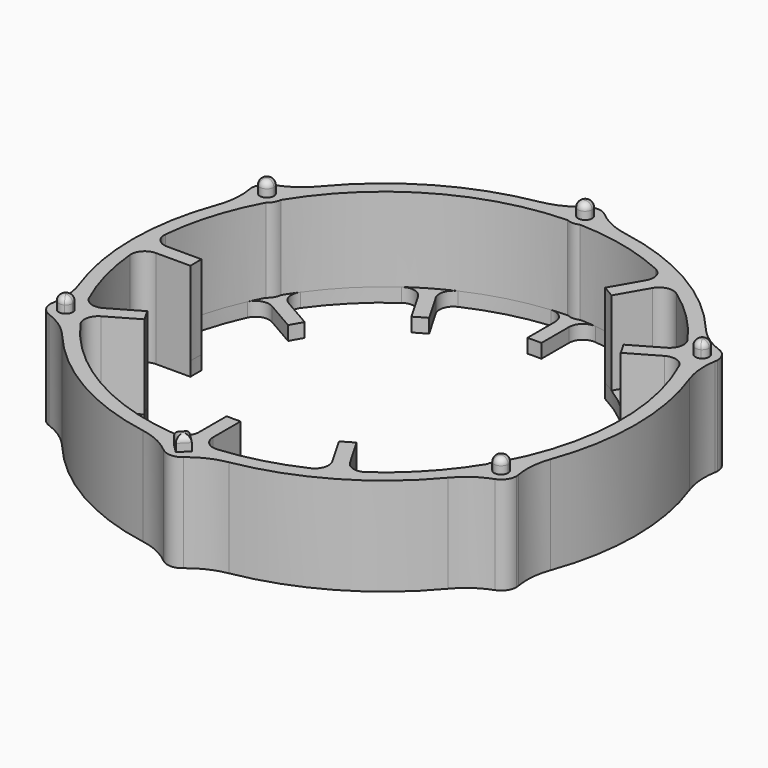
from build123d import *

# Parameters (mm, degrees)
F1_R         = 18
F1_R_2       = 17
F2_DEPTH     = 7
F3_DEPTH     = 7
F4_DEPTH     = 1
F6_DEPTH     = 7
F7_R         = 1
F8_R         = 5
F9_DEPTH     = 8
F10_R        = 0.44999
F11_DEPTH    = 1.8
F12_R        = 13.47
F13_DEPTH    = 1
F14_DEPTH    = 1
F15_T1_DEPTH = 3.7395798703
F15_T3_DEPTH = 1


# Not quite as in the source:
# - a fillet or chamfer that OpenCascade refuses, or shapes differently, is made with other operations: its cross-section is extruded or revolved along the edge and cut away or added
# - a fillet or chamfer is up to 0.001 mm smaller than in the source, because OpenCascade refuses the exact size
# - after a boolean that leaves OpenCascade's solid faulty, fix() repairs it


with BuildPart() as f2:
    # F1 (on Top) → F2 (new body)
    with BuildSketch(Plane.XY):
        Circle(F1_R)
        Circle(F1_R_2, mode=Mode.SUBTRACT)
    extrude(amount=F2_DEPTH)

    # F0 (on Top) → F3 (join)
    with BuildSketch(Plane.XY):
        with BuildLine():
            Line((7.1633711619, 11.4073228059), (8.9293354359, 14.4660626528))
            ThreePointArc((8.9293354359, 14.4660626528), (8.5, 14.7224318643), (8.0633100321, 14.9660626528))
            Line((8.0633100321, 14.9660626528), (6.2973457581, 11.9073228059))
            ThreePointArc((6.2973457581, 11.9073228059), (6.735, 11.665362189), (7.1633711619, 11.4073228059))
        make_face()
        with BuildLine():
            ThreePointArc((-0.5, -16.992645468), (0, -17), (0.5, -16.992645468))
            Line((0.5, -16.992645468), (0.5, -13.46071692))
            ThreePointArc((0.5, -13.46071692), (0, -13.47), (-0.5, -13.46071692))
            Line((-0.5, -13.46071692), (-0.5, -16.992645468))
        make_face()
        with BuildLine():
            ThreePointArc((-14.9660626528, -8.0633100321), (-14.7224318643, -8.5), (-14.4660626528, -8.9293354359))
            Line((-14.4660626528, -8.9293354359), (-11.4073228059, -7.1633711619))
            ThreePointArc((-11.4073228059, -7.1633711619), (-11.665362189, -6.735), (-11.9073228059, -6.2973457581))
            Line((-11.9073228059, -6.2973457581), (-14.9660626528, -8.0633100321))
        make_face()
        with BuildLine():
            Line((11.9073228059, 6.2973457581), (14.9660626528, 8.0633100321))
            ThreePointArc((14.9660626528, 8.0633100321), (14.7224318643, 8.5), (14.4660626528, 8.9293354359))
            Line((14.4660626528, 8.9293354359), (11.4073228059, 7.1633711619))
            ThreePointArc((11.4073228059, 7.1633711619), (11.665362189, 6.735), (11.9073228059, 6.2973457581))
        make_face()
        with BuildLine():
            ThreePointArc((8.0633100321, -14.9660626528), (8.5, -14.7224318643), (8.9293354359, -14.4660626528))
            Line((8.9293354359, -14.4660626528), (7.1633711619, -11.4073228059))
            ThreePointArc((7.1633711619, -11.4073228059), (6.735, -11.665362189), (6.2973457581, -11.9073228059))
            Line((6.2973457581, -11.9073228059), (8.0633100321, -14.9660626528))
        make_face()
        with BuildLine():
            Line((-13.46071692, 0.5), (-16.992645468, 0.5))
            ThreePointArc((-16.992645468, 0.5), (-17, 0), (-16.992645468, -0.5))
            Line((-16.992645468, -0.5), (-13.46071692, -0.5))
            ThreePointArc((-13.46071692, -0.5), (-13.47, 0), (-13.46071692, 0.5))
        make_face()
    extrude(amount=F3_DEPTH)

    # F1 (on Top) → F4 (join)
    with BuildSketch(Plane.XY):
        Circle(F1_R)
        Circle(F1_R_2, mode=Mode.SUBTRACT)
        Circle(F1_R_2)
    extrude(amount=F4_DEPTH)

    # F5 (on Top) → F6 (join)
    with BuildSketch(Plane.XY):
        with BuildLine():
            ThreePointArc((-14.4884572681, 9), (-14.6275367743, 9.5353800561), (-15.0096060035, 9.935377578))
            ThreePointArc((-15.0096060035, 9.935377578), (-15.1731450826, 9.6837837802), (-15.3324673166, 9.4294987133))
            ThreePointArc((-15.3324673166, 9.4294987133), (-15.153718855, 9.2469868663), (-15.0884572681, 9))
            ThreePointArc((-15.0884572681, 9), (-15.3354561915, 8.5687338928), (-15.832419089, 8.5635568422))
            ThreePointArc((-15.832419089, 8.5635568422), (-15.9729752997, 8.2984372068), (-16.1090923805, 8.0310113108))
            ThreePointArc((-16.1090923805, 8.0310113108), (-15.0239657375, 8.0558870238), (-14.4884572681, 9))
        make_face()
        with BuildLine():
            ThreePointArc((-15.3324673166, 9.4294987133), (-15.1731450826, 9.6837837802), (-15.0096060035, 9.935377578))
            ThreePointArc((-15.0096060035, 9.935377578), (-16.5410852123, 9.55), (-16.1090923805, 8.0310113108))
            ThreePointArc((-16.1090923805, 8.0310113108), (-15.9729752997, 8.2984372068), (-15.832419089, 8.5635568422))
            ThreePointArc((-15.832419089, 8.5635568422), (-16.02146997, 9.25), (-15.3324673166, 9.4294987133))
        make_face()
        with BuildLine():
            ThreePointArc((-1.099486377, 17.9663888889), (0, 16.9), (1.099486377, 17.9663888889))
            ThreePointArc((1.099486377, 17.9663888889), (0.7998302171, 17.982220987), (0.4999517724, 17.9930555556))
            ThreePointArc((0.4999517724, 17.9930555556), (0, 17.5), (-0.4999517724, 17.9930555556))
            ThreePointArc((-0.4999517724, 17.9930555556), (-0.7998302171, 17.982220987), (-1.099486377, 17.9663888889))
        make_face()
        with BuildLine():
            ThreePointArc((0.4999517724, 17.9930555556), (0.7998302171, 17.982220987), (1.099486377, 17.9663888889))
            ThreePointArc((1.099486377, 17.9663888889), (1.0998715868, 17.9831924823), (1.1, 18))
            ThreePointArc((1.1, 18), (-0.0168075177, 19.0998715868), (-1.099486377, 17.9663888889))
            ThreePointArc((-1.099486377, 17.9663888889), (-0.7998302171, 17.982220987), (-0.4999517724, 17.9930555556))
            ThreePointArc((-0.4999517724, 17.9930555556), (-0.003472306, 18.4999879429), (0.5, 18))
            ThreePointArc((0.5, 18), (0.4999879429, 17.996527694), (0.4999517724, 17.9930555556))
        make_face()
        with BuildLine():
            ThreePointArc((15.832419089, 8.5635568422), (15.9729752997, 8.2984372068), (16.1090923805, 8.0310113108))
            ThreePointArc((16.1090923805, 8.0310113108), (16.5325702443, 8.4355084694), (16.6884572681, 9))
            ThreePointArc((16.6884572681, 9), (16.1238373242, 9.9609204939), (15.0096060035, 9.935377578))
            ThreePointArc((15.0096060035, 9.935377578), (15.1731450826, 9.6837837802), (15.3324673166, 9.4294987133))
            ThreePointArc((15.3324673166, 9.4294987133), (15.8354441344, 9.4347384132), (16.0884572681, 9))
            ThreePointArc((16.0884572681, 9), (16.0197233753, 8.7469989234), (15.832419089, 8.5635568422))
        make_face()
        with BuildLine():
            ThreePointArc((15.0096060035, 9.935377578), (14.635829324, 8.45), (16.1090923805, 8.0310113108))
            ThreePointArc((16.1090923805, 8.0310113108), (15.9729752997, 8.2984372068), (15.832419089, 8.5635568422))
            ThreePointArc((15.832419089, 8.5635568422), (15.1554445662, 8.75), (15.3324673166, 9.4294987133))
            ThreePointArc((15.3324673166, 9.4294987133), (15.1731450826, 9.6837837802), (15.0096060035, 9.935377578))
        make_face()
        with BuildLine():
            ThreePointArc((-15.3324673166, -9.4294987133), (-15.1731450826, -9.6837837802), (-15.0096060035, -9.935377578))
            ThreePointArc((-15.0096060035, -9.935377578), (-14.6275367743, -9.5353800561), (-14.4884572681, -9))
            ThreePointArc((-14.4884572681, -9), (-15.0239657375, -8.0558870238), (-16.1090923805, -8.0310113108))
            ThreePointArc((-16.1090923805, -8.0310113108), (-15.9729752997, -8.2984372068), (-15.832419089, -8.5635568422))
            ThreePointArc((-15.832419089, -8.5635568422), (-15.3354561915, -8.5687338928), (-15.0884572681, -9))
            ThreePointArc((-15.0884572681, -9), (-15.153718855, -9.2469868663), (-15.3324673166, -9.4294987133))
        make_face()
        with BuildLine():
            ThreePointArc((-16.1090923805, -8.0310113108), (-16.5410852123, -9.55), (-15.0096060035, -9.935377578))
            ThreePointArc((-15.0096060035, -9.935377578), (-15.1731450826, -9.6837837802), (-15.3324673166, -9.4294987133))
            ThreePointArc((-15.3324673166, -9.4294987133), (-16.02146997, -9.25), (-15.832419089, -8.5635568422))
            ThreePointArc((-15.832419089, -8.5635568422), (-15.9729752997, -8.2984372068), (-16.1090923805, -8.0310113108))
        make_face()
        with BuildLine():
            ThreePointArc((0.6255239257, -17.9891278226), (0.8625800837, -17.9793202207), (1.099486377, -17.9663888889))
            ThreePointArc((1.099486377, -17.9663888889), (0, -16.9), (-1.099486377, -17.9663888889))
            ThreePointArc((-1.099486377, -17.9663888889), (-0.8625800837, -17.9793202207), (-0.6255239257, -17.9891278226))
            Line((-0.6255239257, -17.9891278226), (0, -17.3636038969))
            Line((0, -17.3636038969), (0.6255239257, -17.9891278226))
        make_face()
        with BuildLine():
            ThreePointArc((1.1, -18), (1.0998715868, -17.9831924823), (1.099486377, -17.9663888889))
            ThreePointArc((1.099486377, -17.9663888889), (0.8625800837, -17.9793202207), (0.6255239257, -17.9891278226))
            Line((0.6255239257, -17.9891278226), (0.6363961031, -18))
            Line((0.6363961031, -18), (0, -18.6363961031))
            Line((0, -18.6363961031), (-0.6363961031, -18))
            Line((-0.6363961031, -18), (-0.6255239257, -17.9891278226))
            ThreePointArc((-0.6255239257, -17.9891278226), (-0.8625800837, -17.9793202207), (-1.099486377, -17.9663888889))
            ThreePointArc((-1.099486377, -17.9663888889), (-0.0168075177, -19.0998715868), (1.1, -18))
        make_face()
        with BuildLine():
            ThreePointArc((16.6884572681, -9), (16.5325702443, -8.4355084694), (16.1090923805, -8.0310113108))
            ThreePointArc((16.1090923805, -8.0310113108), (15.9729752997, -8.2984372068), (15.832419089, -8.5635568422))
            ThreePointArc((15.832419089, -8.5635568422), (16.0197233753, -8.7469989234), (16.0884572681, -9))
            ThreePointArc((16.0884572681, -9), (15.8354441344, -9.4347384132), (15.3324673166, -9.4294987133))
            ThreePointArc((15.3324673166, -9.4294987133), (15.1731450826, -9.6837837802), (15.0096060035, -9.935377578))
            ThreePointArc((15.0096060035, -9.935377578), (16.1238373242, -9.9609204939), (16.6884572681, -9))
        make_face()
        with BuildLine():
            ThreePointArc((15.832419089, -8.5635568422), (15.9729752997, -8.2984372068), (16.1090923805, -8.0310113108))
            ThreePointArc((16.1090923805, -8.0310113108), (14.635829324, -8.45), (15.0096060035, -9.935377578))
            ThreePointArc((15.0096060035, -9.935377578), (15.1731450826, -9.6837837802), (15.3324673166, -9.4294987133))
            ThreePointArc((15.3324673166, -9.4294987133), (15.1554445662, -8.75), (15.832419089, -8.5635568422))
        make_face()
        with BuildLine():
            ThreePointArc((-15.0884572681, 9), (-15.153718855, 9.2469868663), (-15.3324673166, 9.4294987133))
            ThreePointArc((-15.3324673166, 9.4294987133), (-15.5884572681, 9), (-15.832419089, 8.5635568422))
            ThreePointArc((-15.832419089, 8.5635568422), (-15.3354561915, 8.5687338928), (-15.0884572681, 9))
        make_face()
        with BuildLine():
            ThreePointArc((-15.832419089, 8.5635568422), (-15.5884572681, 9), (-15.3324673166, 9.4294987133))
            ThreePointArc((-15.3324673166, 9.4294987133), (-16.02146997, 9.25), (-15.832419089, 8.5635568422))
        make_face()
        with BuildLine():
            ThreePointArc((-0.4999517724, 17.9930555556), (0, 18), (0.4999517724, 17.9930555556))
            ThreePointArc((0.4999517724, 17.9930555556), (0.4999879429, 17.996527694), (0.5, 18))
            ThreePointArc((0.5, 18), (-0.003472306, 18.4999879429), (-0.4999517724, 17.9930555556))
        make_face()
        with BuildLine():
            ThreePointArc((-0.4999517724, 17.9930555556), (0, 17.5), (0.4999517724, 17.9930555556))
            ThreePointArc((0.4999517724, 17.9930555556), (0, 18), (-0.4999517724, 17.9930555556))
        make_face()
        with BuildLine():
            ThreePointArc((15.3324673166, 9.4294987133), (15.5884572681, 9), (15.832419089, 8.5635568422))
            ThreePointArc((15.832419089, 8.5635568422), (16.0197233753, 8.7469989234), (16.0884572681, 9))
            ThreePointArc((16.0884572681, 9), (15.8354441344, 9.4347384132), (15.3324673166, 9.4294987133))
        make_face()
        with BuildLine():
            ThreePointArc((15.3324673166, 9.4294987133), (15.1554445662, 8.75), (15.832419089, 8.5635568422))
            ThreePointArc((15.832419089, 8.5635568422), (15.5884572681, 9), (15.3324673166, 9.4294987133))
        make_face()
        with BuildLine():
            ThreePointArc((16.0884572681, -9), (16.0197233753, -8.7469989234), (15.832419089, -8.5635568422))
            ThreePointArc((15.832419089, -8.5635568422), (15.5884572681, -9), (15.3324673166, -9.4294987133))
            ThreePointArc((15.3324673166, -9.4294987133), (15.8354441344, -9.4347384132), (16.0884572681, -9))
        make_face()
        with BuildLine():
            ThreePointArc((15.3324673166, -9.4294987133), (15.5884572681, -9), (15.832419089, -8.5635568422))
            ThreePointArc((15.832419089, -8.5635568422), (15.1554445662, -8.75), (15.3324673166, -9.4294987133))
        make_face()
        with BuildLine():
            Line((0.6363961031, -18), (0.6255239257, -17.9891278226))
            ThreePointArc((0.6255239257, -17.9891278226), (0, -18), (-0.6255239257, -17.9891278226))
            Line((-0.6255239257, -17.9891278226), (-0.6363961031, -18))
            Line((-0.6363961031, -18), (0, -18.6363961031))
            Line((0, -18.6363961031), (0.6363961031, -18))
        make_face()
        with BuildLine():
            ThreePointArc((-15.832419089, -8.5635568422), (-16.02146997, -9.25), (-15.3324673166, -9.4294987133))
            ThreePointArc((-15.3324673166, -9.4294987133), (-15.5884572681, -9), (-15.832419089, -8.5635568422))
        make_face()
        with BuildLine():
            ThreePointArc((-15.832419089, -8.5635568422), (-15.5884572681, -9), (-15.3324673166, -9.4294987133))
            ThreePointArc((-15.3324673166, -9.4294987133), (-15.153718855, -9.2469868663), (-15.0884572681, -9))
            ThreePointArc((-15.0884572681, -9), (-15.3354561915, -8.5687338928), (-15.832419089, -8.5635568422))
        make_face()
        with BuildLine():
            ThreePointArc((-0.6255239257, -17.9891278226), (0, -18), (0.6255239257, -17.9891278226))
            Line((0.6255239257, -17.9891278226), (0, -17.3636038969))
            Line((0, -17.3636038969), (-0.6255239257, -17.9891278226))
        make_face()
    extrude(amount=F6_DEPTH)

    # F7
    f7_edges = [f2.edges().sort_by_distance(p)[0] for p in [
        (0.5, -16.992645, 4),
        (8.06331, 14.966063, 4),
        (-14.966063, -8.06331, 4),
        (-16.992645, 0.5, 4),
        (8.929335, -14.466063, 4),
        (-0.5, -16.992645, 4),
        (14.466063, 8.929335, 4),
        (-16.992645, -0.5, 4),
        (8.06331, -14.966063, 4),
        (-14.466063, -8.929335, 4),
        (8.929335, 14.466063, 4),
        (14.966063, 8.06331, 4),
    ]]
    fillet(f7_edges, radius=F7_R)

    # F8 (call 1 of 12: OpenCascade refuses the feature's edges together)
    f8_edges = [f2.edges().sort_by_distance(p)[0] for p in [
        (-16.109092, 8.031011, 3.5),
    ]]
    fillet(f8_edges, radius=F8_R)

    # F8#2 (call 2 of 12)
    f8_2_edges = [f2.edges().sort_by_distance(p)[0] for p in [
        (-15.009606, 9.935378, 3.5),
    ]]
    fillet(f8_2_edges, radius=F8_R)

    # F8#3 (call 3 of 12)
    f8_3_edges = [f2.edges().sort_by_distance(p)[0] for p in [
        (-1.099486, 17.966389, 3.5),
    ]]
    fillet(f8_3_edges, radius=F8_R)

    # F8#4 (call 4 of 12)
    f8_4_edges = [f2.edges().sort_by_distance(p)[0] for p in [
        (1.099486, 17.966389, 3.5),
    ]]
    fillet(f8_4_edges, radius=F8_R)

    # F8#5 (call 5 of 12)
    f8_5_edges = [f2.edges().sort_by_distance(p)[0] for p in [
        (-15.009606, -9.935378, 3.5),
    ]]
    fillet(f8_5_edges, radius=F8_R)

    # F8#6 (call 6 of 12)
    f8_6_edges = [f2.edges().sort_by_distance(p)[0] for p in [
        (-16.109092, -8.031011, 3.5),
    ]]
    fillet(f8_6_edges, radius=F8_R)

    # F8#7 (call 7 of 12)
    f8_7_edges = [f2.edges().sort_by_distance(p)[0] for p in [
        (1.099486, -17.966389, 3.5),
    ]]
    fillet(f8_7_edges, radius=F8_R)

    # F8#8 (call 8 of 12)
    f8_8_edges = [f2.edges().sort_by_distance(p)[0] for p in [
        (-1.099486, -17.966389, 3.5),
    ]]
    fillet(f8_8_edges, radius=F8_R)

    # F8#10 (call 9 of 12)
    f8_10_edges = [f2.edges().sort_by_distance(p)[0] for p in [
        (15.009606, -9.935378, 3.5),
    ]]
    fillet(f8_10_edges, radius=F8_R)

    # F8#11 (call 10 of 12)
    f8_11_edges = [f2.edges().sort_by_distance(p)[0] for p in [
        (16.109092, 8.031011, 3.5),
    ]]
    fillet(f8_11_edges, radius=F8_R)

    # F8#12 (call 11 of 12)
    f8_12_edges = [f2.edges().sort_by_distance(p)[0] for p in [
        (15.009606, 9.935378, 3.5),
    ]]
    fillet(f8_12_edges, radius=F8_R)

    # F8#9 (call 12 of 12)
    f8_9_edges = [f2.edges().sort_by_distance(p)[0] for p in [
        (16.109092, -8.031011, 3.5),
    ]]
    fillet(f8_9_edges, radius=F8_R)

    # F5 (on Top) → F9 (join)
    with BuildSketch(Plane.XY):
        with BuildLine():
            ThreePointArc((-15.832419089, 8.5635568422), (-15.5884572681, 9), (-15.3324673166, 9.4294987133))
            ThreePointArc((-15.3324673166, 9.4294987133), (-16.02146997, 9.25), (-15.832419089, 8.5635568422))
        make_face()
        with BuildLine():
            ThreePointArc((-15.0884572681, 9), (-15.153718855, 9.2469868663), (-15.3324673166, 9.4294987133))
            ThreePointArc((-15.3324673166, 9.4294987133), (-15.5884572681, 9), (-15.832419089, 8.5635568422))
            ThreePointArc((-15.832419089, 8.5635568422), (-15.3354561915, 8.5687338928), (-15.0884572681, 9))
        make_face()
        with BuildLine():
            ThreePointArc((-0.4999517724, 17.9930555556), (0, 18), (0.4999517724, 17.9930555556))
            ThreePointArc((0.4999517724, 17.9930555556), (0.4999879429, 17.996527694), (0.5, 18))
            ThreePointArc((0.5, 18), (-0.003472306, 18.4999879429), (-0.4999517724, 17.9930555556))
        make_face()
        with BuildLine():
            ThreePointArc((-0.4999517724, 17.9930555556), (0, 17.5), (0.4999517724, 17.9930555556))
            ThreePointArc((0.4999517724, 17.9930555556), (0, 18), (-0.4999517724, 17.9930555556))
        make_face()
        with BuildLine():
            ThreePointArc((15.3324673166, 9.4294987133), (15.1554445662, 8.75), (15.832419089, 8.5635568422))
            ThreePointArc((15.832419089, 8.5635568422), (15.5884572681, 9), (15.3324673166, 9.4294987133))
        make_face()
        with BuildLine():
            ThreePointArc((15.3324673166, 9.4294987133), (15.5884572681, 9), (15.832419089, 8.5635568422))
            ThreePointArc((15.832419089, 8.5635568422), (16.0197233753, 8.7469989234), (16.0884572681, 9))
            ThreePointArc((16.0884572681, 9), (15.8354441344, 9.4347384132), (15.3324673166, 9.4294987133))
        make_face()
        with BuildLine():
            ThreePointArc((15.3324673166, -9.4294987133), (15.5884572681, -9), (15.832419089, -8.5635568422))
            ThreePointArc((15.832419089, -8.5635568422), (15.1554445662, -8.75), (15.3324673166, -9.4294987133))
        make_face()
        with BuildLine():
            ThreePointArc((16.0884572681, -9), (16.0197233753, -8.7469989234), (15.832419089, -8.5635568422))
            ThreePointArc((15.832419089, -8.5635568422), (15.5884572681, -9), (15.3324673166, -9.4294987133))
            ThreePointArc((15.3324673166, -9.4294987133), (15.8354441344, -9.4347384132), (16.0884572681, -9))
        make_face()
        with BuildLine():
            Line((0.6363961031, -18), (0.6255239257, -17.9891278226))
            ThreePointArc((0.6255239257, -17.9891278226), (0, -18), (-0.6255239257, -17.9891278226))
            Line((-0.6255239257, -17.9891278226), (-0.6363961031, -18))
            Line((-0.6363961031, -18), (0, -18.6363961031))
            Line((0, -18.6363961031), (0.6363961031, -18))
        make_face()
        with BuildLine():
            ThreePointArc((-0.6255239257, -17.9891278226), (0, -18), (0.6255239257, -17.9891278226))
            Line((0.6255239257, -17.9891278226), (0, -17.3636038969))
            Line((0, -17.3636038969), (-0.6255239257, -17.9891278226))
        make_face()
        with BuildLine():
            ThreePointArc((-15.832419089, -8.5635568422), (-16.02146997, -9.25), (-15.3324673166, -9.4294987133))
            ThreePointArc((-15.3324673166, -9.4294987133), (-15.5884572681, -9), (-15.832419089, -8.5635568422))
        make_face()
        with BuildLine():
            ThreePointArc((-15.832419089, -8.5635568422), (-15.5884572681, -9), (-15.3324673166, -9.4294987133))
            ThreePointArc((-15.3324673166, -9.4294987133), (-15.153718855, -9.2469868663), (-15.0884572681, -9))
            ThreePointArc((-15.0884572681, -9), (-15.3354561915, -8.5687338928), (-15.832419089, -8.5635568422))
        make_face()
    extrude(amount=F9_DEPTH)

    # F10 (radius 0.45 in the source; OpenCascade refuses exactly that, so slightly less here)
    f10_edges = [f2.edges().sort_by_distance(p)[0] for p in [
        (-15.844447, -8.570501, 8),
        (-15.344495, 9.436443, 8),
        (0.499952, 18.006944, 8),
        (15.344495, 9.436443, 8),
        (15.844447, -8.570501, 8),
        (0.318198, -17.681802, 8),
        (-0.318198, -18.318198, 8),
        (0.318198, -18.318198, 8),
        (-0.318198, -17.681802, 8),
    ]]
    fillet(f10_edges, radius=F10_R)

    # F5 (on Top) → F11 (cut)
    with BuildSketch(Plane.XY):
        with BuildLine():
            ThreePointArc((-15.832419089, -8.5635568422), (-16.02146997, -9.25), (-15.3324673166, -9.4294987133))
            ThreePointArc((-15.3324673166, -9.4294987133), (-15.5884572681, -9), (-15.832419089, -8.5635568422))
        make_face()
        with BuildLine():
            ThreePointArc((-15.832419089, -8.5635568422), (-15.5884572681, -9), (-15.3324673166, -9.4294987133))
            ThreePointArc((-15.3324673166, -9.4294987133), (-15.153718855, -9.2469868663), (-15.0884572681, -9))
            ThreePointArc((-15.0884572681, -9), (-15.3354561915, -8.5687338928), (-15.832419089, -8.5635568422))
        make_face()
        with BuildLine():
            Line((0.6363961031, -18), (0.6255239257, -17.9891278226))
            ThreePointArc((0.6255239257, -17.9891278226), (0, -18), (-0.6255239257, -17.9891278226))
            Line((-0.6255239257, -17.9891278226), (-0.6363961031, -18))
            Line((-0.6363961031, -18), (0, -18.6363961031))
            Line((0, -18.6363961031), (0.6363961031, -18))
        make_face()
        with BuildLine():
            ThreePointArc((-0.6255239257, -17.9891278226), (0, -18), (0.6255239257, -17.9891278226))
            Line((0.6255239257, -17.9891278226), (0, -17.3636038969))
            Line((0, -17.3636038969), (-0.6255239257, -17.9891278226))
        make_face()
        with BuildLine():
            ThreePointArc((15.3324673166, -9.4294987133), (15.5884572681, -9), (15.832419089, -8.5635568422))
            ThreePointArc((15.832419089, -8.5635568422), (15.1554445662, -8.75), (15.3324673166, -9.4294987133))
        make_face()
        with BuildLine():
            ThreePointArc((16.0884572681, -9), (16.0197233753, -8.7469989234), (15.832419089, -8.5635568422))
            ThreePointArc((15.832419089, -8.5635568422), (15.5884572681, -9), (15.3324673166, -9.4294987133))
            ThreePointArc((15.3324673166, -9.4294987133), (15.8354441344, -9.4347384132), (16.0884572681, -9))
        make_face()
        with BuildLine():
            ThreePointArc((15.3324673166, 9.4294987133), (15.1554445662, 8.75), (15.832419089, 8.5635568422))
            ThreePointArc((15.832419089, 8.5635568422), (15.5884572681, 9), (15.3324673166, 9.4294987133))
        make_face()
        with BuildLine():
            ThreePointArc((15.3324673166, 9.4294987133), (15.5884572681, 9), (15.832419089, 8.5635568422))
            ThreePointArc((15.832419089, 8.5635568422), (16.0197233753, 8.7469989234), (16.0884572681, 9))
            ThreePointArc((16.0884572681, 9), (15.8354441344, 9.4347384132), (15.3324673166, 9.4294987133))
        make_face()
        with BuildLine():
            ThreePointArc((-0.4999517724, 17.9930555556), (0, 17.5), (0.4999517724, 17.9930555556))
            ThreePointArc((0.4999517724, 17.9930555556), (0, 18), (-0.4999517724, 17.9930555556))
        make_face()
        with BuildLine():
            ThreePointArc((-0.4999517724, 17.9930555556), (0, 18), (0.4999517724, 17.9930555556))
            ThreePointArc((0.4999517724, 17.9930555556), (0.4999879429, 17.996527694), (0.5, 18))
            ThreePointArc((0.5, 18), (-0.003472306, 18.4999879429), (-0.4999517724, 17.9930555556))
        make_face()
        with BuildLine():
            ThreePointArc((-15.832419089, 8.5635568422), (-15.5884572681, 9), (-15.3324673166, 9.4294987133))
            ThreePointArc((-15.3324673166, 9.4294987133), (-16.02146997, 9.25), (-15.832419089, 8.5635568422))
        make_face()
        with BuildLine():
            ThreePointArc((-15.0884572681, 9), (-15.153718855, 9.2469868663), (-15.3324673166, 9.4294987133))
            ThreePointArc((-15.3324673166, 9.4294987133), (-15.5884572681, 9), (-15.832419089, 8.5635568422))
            ThreePointArc((-15.832419089, 8.5635568422), (-15.3354561915, 8.5687338928), (-15.0884572681, 9))
        make_face()
    extrude(amount=F11_DEPTH, mode=Mode.SUBTRACT)

    # F12 (on Top) → F13 (cut)
    with BuildSketch(Plane.XY):
        Circle(F12_R)
    extrude(amount=F13_DEPTH, mode=Mode.SUBTRACT)

    add(f2.part.fix(), mode=Mode.REPLACE)

    # F0 (on Top) → F14 (cut)
    with BuildSketch(Plane.XY):
        with BuildLine():
            ThreePointArc((8.9293354359, -14.4660626528), (12.0208152802, -12.0208152802), (14.4660626528, -8.9293354359))
            Line((14.4660626528, -8.9293354359), (11.4073228059, -7.1633711619))
            ThreePointArc((11.4073228059, -7.1633711619), (9.5247283426, -9.5247283426), (7.1633711619, -11.4073228059))
            Line((7.1633711619, -11.4073228059), (8.9293354359, -14.4660626528))
        make_face()
        with BuildLine():
            Line((6.2973457581, 11.9073228059), (8.0633100321, 14.9660626528))
            ThreePointArc((8.0633100321, 14.9660626528), (4.3999237667, 16.4207390469), (0.5, 16.992645468))
            Line((0.5, 16.992645468), (0.5, 13.46071692))
            ThreePointArc((0.5, 13.46071692), (3.4862925375, 13.0110208801), (6.2973457581, 11.9073228059))
        make_face()
        with BuildLine():
            ThreePointArc((-8.0633100321, -14.9660626528), (-4.3999237667, -16.4207390469), (-0.5, -16.992645468))
            Line((-0.5, -16.992645468), (-0.5, -13.46071692))
            ThreePointArc((-0.5, -13.46071692), (-3.4862925375, -13.0110208801), (-6.2973457581, -11.9073228059))
            Line((-6.2973457581, -11.9073228059), (-8.0633100321, -14.9660626528))
        make_face()
        with BuildLine():
            Line((-0.5, 13.46071692), (-0.5, 16.992645468))
            ThreePointArc((-0.5, 16.992645468), (-4.3999237667, 16.4207390469), (-8.0633100321, 14.9660626528))
            Line((-8.0633100321, 14.9660626528), (-6.2973457581, 11.9073228059))
            ThreePointArc((-6.2973457581, 11.9073228059), (-3.4862925375, 13.0110208801), (-0.5, 13.46071692))
        make_face()
        with BuildLine():
            Line((-7.1633711619, 11.4073228059), (-8.9293354359, 14.4660626528))
            ThreePointArc((-8.9293354359, 14.4660626528), (-12.0208152802, 12.0208152802), (-14.4660626528, 8.9293354359))
            Line((-14.4660626528, 8.9293354359), (-11.4073228059, 7.1633711619))
            ThreePointArc((-11.4073228059, 7.1633711619), (-9.5247283426, 9.5247283426), (-7.1633711619, 11.4073228059))
        make_face()
        with BuildLine():
            Line((-11.9073228059, 6.2973457581), (-14.9660626528, 8.0633100321))
            ThreePointArc((-14.9660626528, 8.0633100321), (-16.4207390469, 4.3999237667), (-16.992645468, 0.5))
            Line((-16.992645468, 0.5), (-13.46071692, 0.5))
            ThreePointArc((-13.46071692, 0.5), (-13.0110208801, 3.4862925375), (-11.9073228059, 6.2973457581))
        make_face()
        with BuildLine():
            ThreePointArc((-16.992645468, -0.5), (-16.4207390469, -4.3999237667), (-14.9660626528, -8.0633100321))
            Line((-14.9660626528, -8.0633100321), (-11.9073228059, -6.2973457581))
            ThreePointArc((-11.9073228059, -6.2973457581), (-13.0110208801, -3.4862925375), (-13.46071692, -0.5))
            Line((-13.46071692, -0.5), (-16.992645468, -0.5))
        make_face()
    extrude(amount=F14_DEPTH, mode=Mode.SUBTRACT)

    # F15: fillet of radius 1 on 14 edges, made by hand

    # F15_s2 → F15_t1 (join)
    with BuildSketch(Plane.XY):
        with BuildLine():
            ThreePointArc((-15.9295323221, 0.5), (-16.669042295, 0.8268543991), (-16.9251280922, 1.59375))
            ThreePointArc((-16.9251280922, 1.59375), (-16.9677020567, 1.0474191685), (-16.992645468, 0.5))
            Line((-16.992645468, 0.5), (-15.9295323221, 0.5))
        make_face()
        with BuildLine():
            ThreePointArc((-14.0453796613, -7.5317534591), (-14.8492412838, -7.6184442326), (-15.4544658902, -7.0823360588))
            ThreePointArc((-15.4544658902, -7.0823360588), (-15.2181706092, -7.57675942), (-14.9660626528, -8.0633100321))
            Line((-14.9660626528, -8.0633100321), (-14.0453796613, -7.5317534591))
        make_face()
        with BuildLine():
            ThreePointArc((-16.9251280922, -1.59375), (-16.669042295, -0.8268543991), (-15.9295323221, -0.5))
            Line((-15.9295323221, -0.5), (-16.992645468, -0.5))
            ThreePointArc((-16.992645468, -0.5), (-16.9677020567, -1.0474191685), (-16.9251280922, -1.59375))
        make_face()
        with BuildLine():
            ThreePointArc((7.0823360588, 15.4544658902), (7.6184442326, 14.8492412837), (7.5317534591, 14.0453796613))
            Line((7.5317534591, 14.0453796613), (8.0633100321, 14.9660626528))
            ThreePointArc((8.0633100321, 14.9660626528), (7.57675942, 15.2181706092), (7.0823360588, 15.4544658902))
        make_face()
        with BuildLine():
            ThreePointArc((8.3977788629, -13.5453796613), (9.0505980623, -14.0223868846), (9.8427920334, -13.8607158902))
            ThreePointArc((9.8427920334, -13.8607158902), (9.3909426367, -14.1707514407), (8.9293354359, -14.4660626528))
            Line((8.9293354359, -14.4660626528), (8.3977788629, -13.5453796613))
        make_face()
        with BuildLine():
            ThreePointArc((-0.5, -15.9295323221), (-0.8268543991, -16.669042295), (-1.59375, -16.9251280922))
            ThreePointArc((-1.59375, -16.9251280922), (-1.0474191685, -16.9677020567), (-0.5, -16.992645468))
            Line((-0.5, -16.992645468), (-0.5, -15.9295323221))
        make_face()
    extrude(amount=F15_T1_DEPTH)

    # F15_s4 → F15_t3 (join)
    with BuildSketch(Plane.XY):
        with BuildLine():
            ThreePointArc((-7.0823360588, -15.4544658902), (-7.6184442326, -14.8492412837), (-7.5317534591, -14.0453796613))
            Line((-7.5317534591, -14.0453796613), (-8.0633100321, -14.9660626528))
            ThreePointArc((-8.0633100321, -14.9660626528), (-7.57675942, -15.2181706092), (-7.0823360588, -15.4544658902))
        make_face()
        with BuildLine():
            ThreePointArc((-13.8607158902, 9.8427920334), (-14.0223868846, 9.0505980623), (-13.5453796613, 8.3977788629))
            Line((-13.5453796613, 8.3977788629), (-14.4660626528, 8.9293354359))
            ThreePointArc((-14.4660626528, 8.9293354359), (-14.1707514407, 9.3909426367), (-13.8607158902, 9.8427920334))
        make_face()
        with BuildLine():
            ThreePointArc((-7.0823360588, 15.4544658902), (-7.6184442326, 14.8492412837), (-7.5317534591, 14.0453796613))
            Line((-7.5317534591, 14.0453796613), (-8.0633100321, 14.9660626528))
            ThreePointArc((-8.0633100321, 14.9660626528), (-7.57675942, 15.2181706092), (-7.0823360588, 15.4544658902))
        make_face()
        with BuildLine():
            ThreePointArc((-9.8427920334, 13.8607158902), (-9.0505980623, 14.0223868846), (-8.3977788629, 13.5453796613))
            Line((-8.3977788629, 13.5453796613), (-8.9293354359, 14.4660626528))
            ThreePointArc((-8.9293354359, 14.4660626528), (-9.3909426367, 14.1707514407), (-9.8427920334, 13.8607158902))
        make_face()
        with BuildLine():
            ThreePointArc((-1.59375, 16.9251280922), (-0.8268543991, 16.669042295), (-0.5, 15.9295323221))
            Line((-0.5, 15.9295323221), (-0.5, 16.992645468))
            ThreePointArc((-0.5, 16.992645468), (-1.0474191685, 16.9677020567), (-1.59375, 16.9251280922))
        make_face()
        with BuildLine():
            ThreePointArc((13.8607158902, -9.8427920334), (14.0223868846, -9.0505980623), (13.5453796613, -8.3977788629))
            Line((13.5453796613, -8.3977788629), (14.4660626528, -8.9293354359))
            ThreePointArc((14.4660626528, -8.9293354359), (14.1707514407, -9.3909426367), (13.8607158902, -9.8427920334))
        make_face()
        with BuildLine():
            ThreePointArc((-15.4544658902, 7.0823360588), (-14.8492412837, 7.6184442326), (-14.0453796613, 7.5317534591))
            Line((-14.0453796613, 7.5317534591), (-14.9660626528, 8.0633100321))
            ThreePointArc((-14.9660626528, 8.0633100321), (-15.2181706092, 7.57675942), (-15.4544658902, 7.0823360588))
        make_face()
        with BuildLine():
            ThreePointArc((1.59375, 16.9251280922), (0.8268543991, 16.669042295), (0.5, 15.9295323221))
            Line((0.5, 15.9295323221), (0.5, 16.992645468))
            ThreePointArc((0.5, 16.992645468), (1.0474191685, 16.9677020567), (1.59375, 16.9251280922))
        make_face()
    extrude(amount=F15_T3_DEPTH)


solid = f2.part
